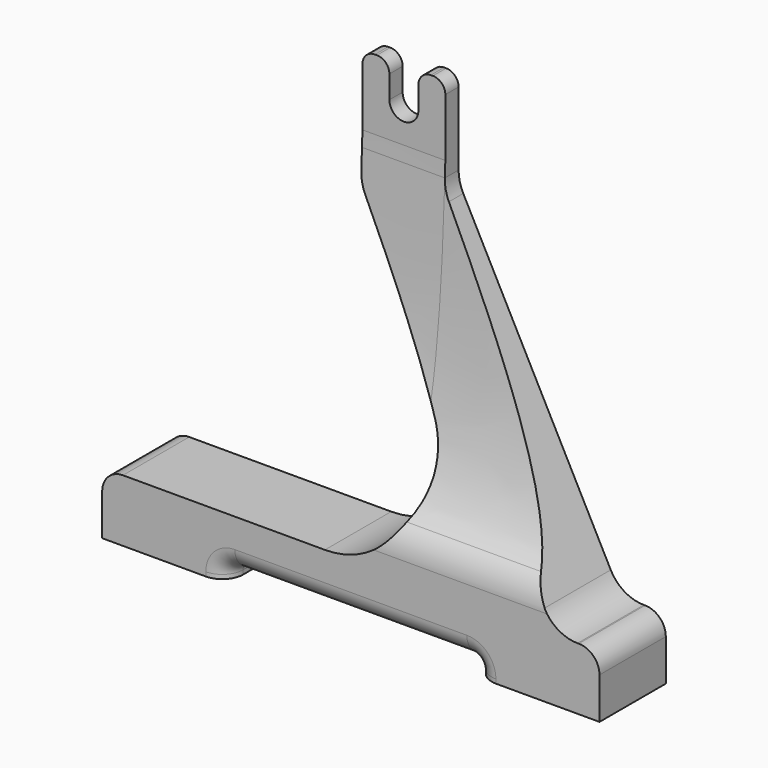
from build123d import *

# Parameters (mm, degrees)
F1_DEPTH    = 20
F3_W        = 25
F3_H        = 15
F4_DEPTH    = 2
F5_DEPTH    = 37.5
F6_T1_DEPTH = 58.6389885579
F7_R        = 5
F8_W        = 5
F8_H        = 5
F9_DEPTH    = 5


# Not quite as in the source:
# - a fillet or chamfer that OpenCascade refuses, or shapes differently, is made with other operations: its cross-section is extruded or revolved along the edge and cut away or added


with BuildPart() as f1:
    # F0 (on Front) → F1 (new body)
    with BuildSketch(Plane.XZ):
        with BuildLine():
            ThreePointArc((3.5, 105), (0, 101.5), (-3.5, 105))
            Line((-3.5, 105), (-3.5, 110.5))
            ThreePointArc((-3.5, 110.5), (-4.3786796564, 112.6213203436), (-6.5, 113.5))
            Line((-6.5, 113.5), (-7, 113.5))
            ThreePointArc((-7, 113.5), (-9.1213203436, 112.6213203436), (-10, 110.5))
            Line((-10, 110.5), (-10, 87.95553398))
            ThreePointArc((-10, 87.95553398), (-9.7135967012, 85.5793944372), (-8.8707921745, 83.339361735))
            Line((-8.8707921745, 83.339361735), (11.4796707875, 44.2323444901))
            ThreePointArc((11.4796707875, 44.2323444901), (10.8355554003, 24.6232685734), (-6.2619135616, 15))
            Line((-6.2619135616, 15), (-20, 15))
            Line((-20, 15), (-55, 15))
            ThreePointArc((-55, 15), (-58.5355339059, 13.5355339059), (-60, 10))
            Line((-60, 10), (-60, 0))
            Line((-60, 0), (-30, 0))
            Line((-30, 0), (-30, 1))
            ThreePointArc((-30, 1), (-29.4142135624, 2.4142135624), (-28, 3))
            Line((-28, 3), (28, 3))
            ThreePointArc((28, 3), (29.4142135624, 2.4142135624), (30, 1))
            Line((30, 1), (30, 0))
            Line((30, 0), (60, 0))
            Line((60, 0), (60, 10))
            ThreePointArc((60, 10), (58.5355339059, 13.5355339059), (55, 15))
            Line((55, 15), (54.6997101643, 15))
            ThreePointArc((54.6997101643, 15), (50.0301810224, 16.3061389672), (46.7159972072, 19.8454449795))
            Line((46.7159972072, 19.8454449795), (11.1292078255, 88.2317607423))
            ThreePointArc((11.1292078255, 88.2317607423), (10.2864032988, 90.4717934444), (10, 92.8479329873))
            Line((10, 92.8479329873), (10, 110.5))
            ThreePointArc((10, 110.5), (9.1213203436, 112.6213203436), (7, 113.5))
            Line((7, 113.5), (6.5, 113.5))
            ThreePointArc((6.5, 113.5), (4.3786796564, 112.6213203436), (3.5, 110.5))
            Line((3.5, 110.5), (3.5, 105))
        make_face()
    extrude(amount=F1_DEPTH)

    # F3 (on face) → F4 (cut)
    with BuildSketch(Plane(origin=(0, 0, 0), x_dir=(1, 0, 0), z_dir=(0, 0, -1))):
        with Locations((-45, 10)):
            Rectangle(F3_W, F3_H)
        with Locations((45, 10)):
            Rectangle(F3_W, F3_H)
    extrude(amount=-F4_DEPTH, mode=Mode.SUBTRACT)

    # F2 (on face) → F5 (cut, symmetric)
    with BuildSketch(Plane.YZ.offset(10)):
        with BuildLine():
            Line((-4, 110.5), (-4, 116.6035970932))
            Line((-4, 116.6035970932), (-20, 116.6035970932))
            Line((-20, 116.6035970932), (-25.1650810242, 116.6035970932))
            Line((-25.1650810242, 116.6035970932), (-25.1650810242, 79.4423669577))
            add(Edge.make_bspline(
                [(-4.1398803615, 92.8479329873), (-5.1496440899, 67.4077745329), (-7.6646247124, 33.6991611835), (-28.2911028311, 14.4998998622), (-25.1674044469, 51.8834188861), (-25.1650810242, 79.4423669577)],
                knots=[0.0193593225, 0.0193593225, 0.0193593225, 0.0193593225, 0.4254603459, 0.6072510197, 1, 1, 1, 1], degree=3))
            Line((-4.1398803615, 92.8479329873), (-20, 92.8479329873))
            Line((-20, 92.8479329873), (-20, 110.5))
            Line((-20, 110.5), (-4, 110.5))
        make_face()
        with BuildLine():
            Line((-4, 96.5), (-4, 110.5))
            Line((-4, 110.5), (-20, 110.5))
            Line((-20, 110.5), (-20, 92.8479329873))
            Line((-20, 92.8479329873), (-4.1398803615, 92.8479329873))
            add(Edge.make_bspline(
                [(-4, 96.5), (-4.0452603939, 95.2783561916), (-4.0917437144, 94.0606958296), (-4.1398803615, 92.8479329873)],
                knots=[0, 0, 0, 0, 0.0193593225, 0.0193593225, 0.0193593225, 0.0193593225], degree=3))
        make_face()
    extrude(amount=F5_DEPTH, both=True, mode=Mode.SUBTRACT)

    # F6: fillet of radius 10 on 2 edges, made by hand

    # F6_s2 → F6_t1 (cut)
    with BuildSketch(Plane.YZ.offset(-1.8596902738)):
        with BuildLine():
            ThreePointArc((-17.2619280984, 25.6086451358), (-19.2905970582, 22.4331187004), (-20.0004, 18.7323558501))
            Line((-20.0004, 18.7323558501), (-21.00064, 18.7323558501))
            ThreePointArc((-21.00064, 18.7323558501), (-21.00024, 21.1277820745), (-21.00024, 23.523208299))
            Line((-21.00024, 23.523208299), (-20.397089154, 24.4412498347))
            ThreePointArc((-20.397089154, 24.4412498347), (-19.1489832388, 25.2196704089), (-17.9883209083, 26.2962740644))
            Line((-17.9883209083, 26.2962740644), (-17.2619280984, 25.6086451358))
        make_face()
    extrude(amount=F6_T1_DEPTH, mode=Mode.SUBTRACT)

    # F7
    f7_edges = [f1.edges().sort_by_distance(p)[0] for p in [
        (0, -20, 3),
        (-30, -20, 0.5),
        (-29.414214, -20, 2.414214),
        (29.414214, -20, 2.414214),
        (30, -20, 0.5),
    ]]
    fillet(f7_edges, radius=F7_R)

    # F8 (on face) → F9 (cut)
    with BuildSketch(Plane.XZ):
        with Locations((52.5, 7.5)):
            Rectangle(F8_W, F8_H)
        with Locations((-52.5, 7.5)):
            Rectangle(F8_W, F8_H)
    extrude(amount=F9_DEPTH, mode=Mode.SUBTRACT)


solid = f1.part
